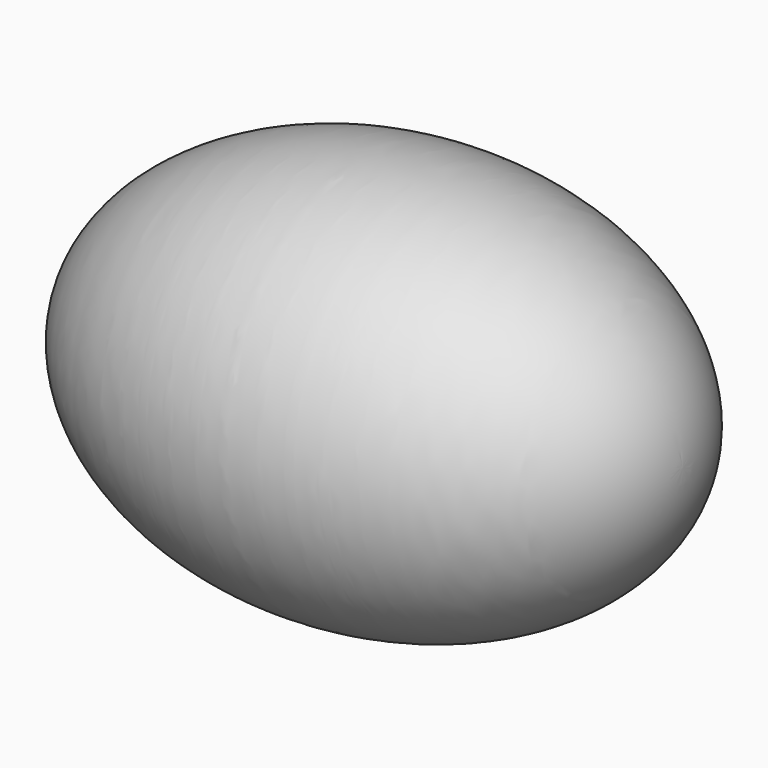
from build123d import *


with BuildPart() as f1:
    # F0 (on Front) → F1 (revolve)
    with BuildSketch(Plane.XZ):
        with BuildLine():
            add(Edge.make_bspline(
                [(39.6005958319, 84.6015363932), (38.9612849501, 92.76215437), (26.5955600586, 91.7934112543), (14.2298351672, 90.8246681387), (14.869146049, 82.6640501618)],
                knots=[0, 0, 0, 1.5707963268, 1.5707963268, 3.1415926536, 3.1415926536, 3.1415926536], degree=2, weights=[1, 0.7071067812, 1, 0.7071067812, 1]))
            Line((14.869146049, 82.6640501618), (39.6005958319, 84.6015363932))
        make_face()
    revolve(axis=Axis((27.2348709404, 0, 83.6327932775), (0.9969453978, 0, 0.0781016883)))


solid = f1.part
